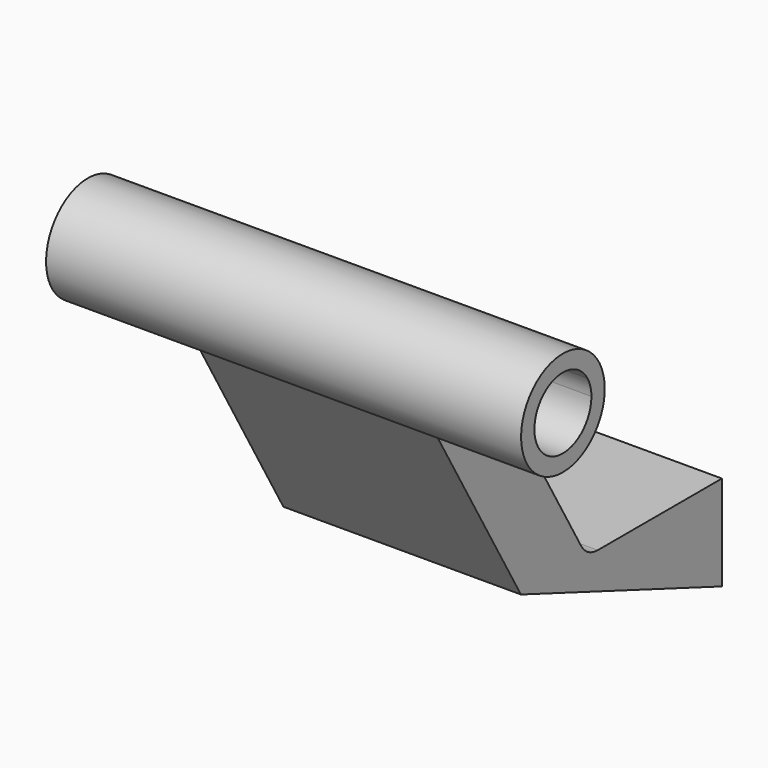
from build123d import *

# Parameters (mm, degrees)
F1_DEPTH = 50
F2_DEPTH = 25
F4_DEPTH = 10
F5_R     = 5


with BuildPart() as f1:
    # F0 (on Right) → F1 (new body, symmetric)
    with BuildSketch(Plane.YZ):
        with BuildLine():
            ThreePointArc((-62.094011, 70), (-79.942732, 78.607846), (-75.565832, 59.28132))
            Line((-75.565832, 59.28132), (-79.589201, 66.25))
            ThreePointArc((-79.589201, 66.25), (-76.844011, 76.495191), (-66.59882, 73.75))
            Line((-66.59882, 73.75), (-62.575451, 66.78132))
            ThreePointArc((-62.575451, 66.78132), (-62.215037, 68.372757), (-62.094011, 70))
        make_face()
        with BuildLine():
            Line((-79.589201, 66.25), (-75.565832, 59.28132))
            ThreePointArc((-75.565832, 59.28132), (-67.594011, 60.473721), (-62.575451, 66.78132))
            Line((-62.575451, 66.78132), (-66.59882, 73.75))
            ThreePointArc((-66.59882, 73.75), (-65.849567, 71.941143), (-65.594011, 70))
            ThreePointArc((-65.594011, 70), (-71.152868, 62.755556), (-79.589201, 66.25))
        make_face()
    extrude(amount=F1_DEPTH, both=True)

    # F0 (on Right) → F2 (join, symmetric)
    with BuildSketch(Plane.YZ):
        with BuildLine():
            Line((-52.886751, 20), (0, 0))
            Line((0, 0), (0, 20))
            Line((0, 20), (-35.566243, 20))
            Line((-35.566243, 20), (-62.575451, 66.78132))
            ThreePointArc((-62.575451, 66.78132), (-67.594011, 60.473721), (-75.565832, 59.28132))
            Line((-75.565832, 59.28132), (-52.886751, 20))
        make_face()
    extrude(amount=F2_DEPTH, both=True)

    # F3 (on Top) → F4 (cut)
    with BuildSketch(Plane.XY):
        with BuildLine():
            ThreePointArc((-7.475, -5), (-10, -7.525), (-12.525, -5))
            Line((-12.525, -5), (-12.525, -30))
            ThreePointArc((-12.525, -30), (-10, -27.475), (-7.475, -30))
            Line((-7.475, -30), (-7.475, -5))
        make_face()
        with BuildLine():
            ThreePointArc((-7.475, -5), (-10, -2.475), (-12.525, -5))
            Line((-12.525, -5), (-7.475, -5))
        make_face()
        with BuildLine():
            Line((-7.475, -5), (-12.525, -5))
            ThreePointArc((-12.525, -5), (-10, -7.525), (-7.475, -5))
        make_face()
        with BuildLine():
            ThreePointArc((-7.475, -30), (-10, -27.475), (-12.525, -30))
            Line((-12.525, -30), (-7.475, -30))
        make_face()
        with BuildLine():
            Line((-7.475, -30), (-12.525, -30))
            ThreePointArc((-12.525, -30), (-10, -32.525), (-7.475, -30))
        make_face()
        with BuildLine():
            ThreePointArc((12.525, -5), (10, -7.525), (7.475, -5))
            Line((7.475, -5), (7.475, -30))
            ThreePointArc((7.475, -30), (10, -27.475), (12.525, -30))
            Line((12.525, -30), (12.525, -5))
        make_face()
        with BuildLine():
            ThreePointArc((12.525, -5), (10, -2.475), (7.475, -5))
            Line((7.475, -5), (12.525, -5))
        make_face()
        with BuildLine():
            Line((12.525, -5), (7.475, -5))
            ThreePointArc((7.475, -5), (10, -7.525), (12.525, -5))
        make_face()
        with BuildLine():
            ThreePointArc((12.525, -30), (10, -27.475), (7.475, -30))
            Line((7.475, -30), (12.525, -30))
        make_face()
        with BuildLine():
            Line((12.525, -30), (7.475, -30))
            ThreePointArc((7.475, -30), (10, -32.525), (12.525, -30))
        make_face()
    extrude(amount=F4_DEPTH, mode=Mode.SUBTRACT)

    # F5
    f5_edges = [f1.edges().sort_by_distance(p)[0] for p in [
        (0, -35.566243, 20),
    ]]
    fillet(f5_edges, radius=F5_R)


solid = f1.part
